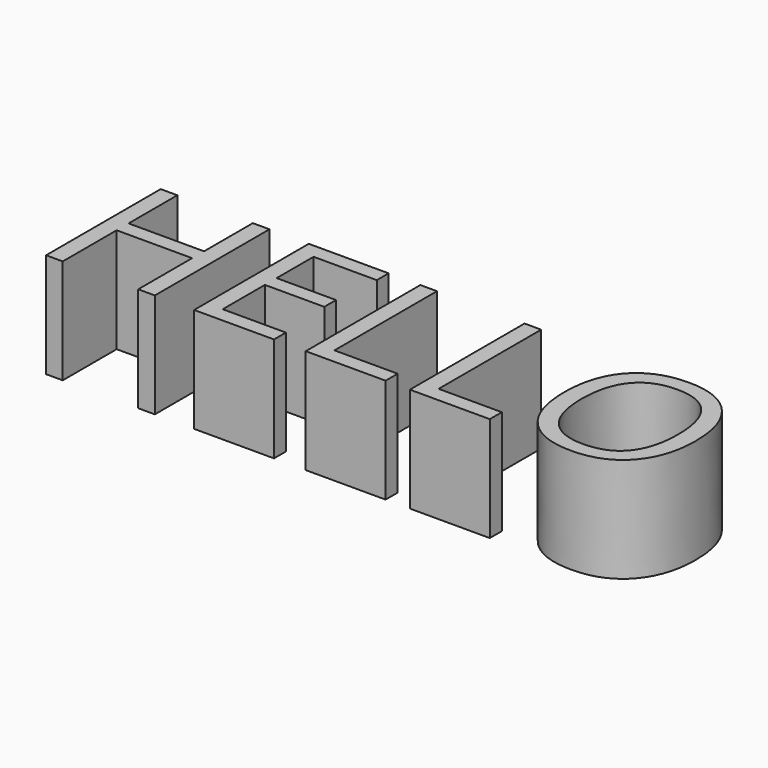
from build123d import *

# Parameters (mm, degrees)
F0_TEXT_SIZE = 48.6801378429
F1_DEPTH     = 25.4


# Not quite as in the source:
# - Text() gives the source's letters only with a copy of the font that has no kerning and outlines rounded to 1/6400 em; it was checked with that copy


with BuildPart() as f1:
    # F0 (on Top) → F1 (new body)
    with BuildSketch(Plane.XY):
        with Locations((-61.6391263902, 21.9967067242)):
            Text('HELLO', F0_TEXT_SIZE, font='Open Sans', text_align=(TextAlign.LEFT, TextAlign.BOTTOM))
    extrude(amount=F1_DEPTH)


with BuildPart() as f1_1:
    # F2: moved
    add(f1.part.moved(Location((-13.716, -2.032, 0))))


solid = f1_1.part
